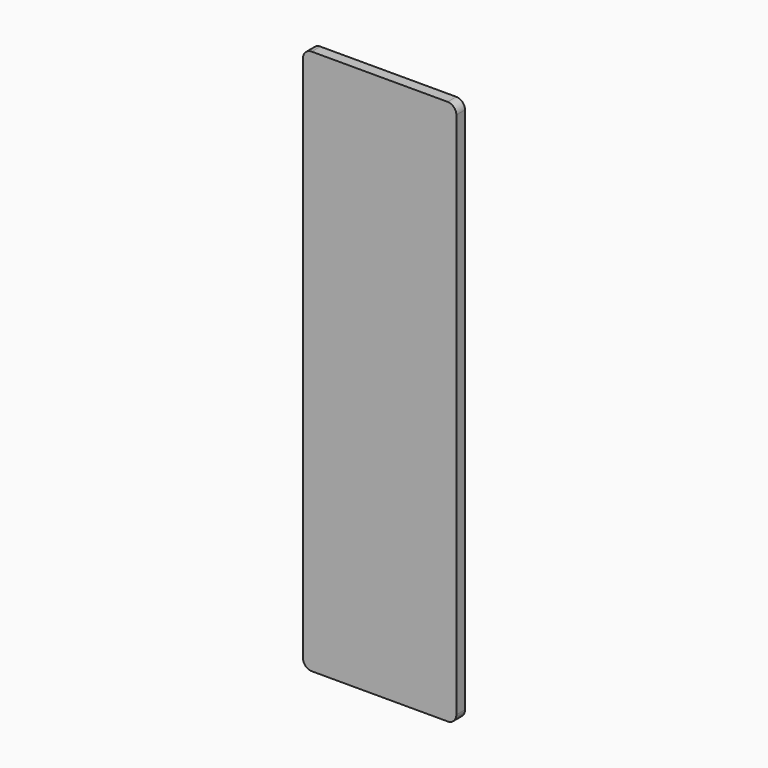
from build123d import *

# Parameters (mm, degrees)
F1_DEPTH = 3.175


# Not quite as in the source:
# - a length typed as a fraction of an inch, garbled in the dataset ("3 / 203.2 mm" for 3/8 in), is restored


with BuildPart() as f1:
    # F0 (on Front) → F1 (new body)
    with BuildSketch(Plane.XZ):
        with BuildLine():
            Line((21.49735579, 94.8843865406), (-18.12664421, 94.8843865406))
            ThreePointArc((-18.12664421, 94.8843865406), (-19.9226954343, 94.1404377648), (-20.66664421, 92.3443865406))
            Line((-20.66664421, 92.3443865406), (-20.66664421, -61.5796134594))
            ThreePointArc((-20.66664421, -61.5796134594), (-19.9226954343, -63.3756646836), (-18.12664421, -64.1196134594))
            Line((-18.12664421, -64.1196134594), (21.49735579, -64.1196134594))
            ThreePointArc((21.49735579, -64.1196134594), (23.2934070142, -63.3756646836), (24.03735579, -61.5796134594))
            Line((24.03735579, -61.5796134594), (24.03735579, 92.3443865406))
            ThreePointArc((24.03735579, 92.3443865406), (23.2934070142, 94.1404377648), (21.49735579, 94.8843865406))
        make_face()
    extrude(amount=F1_DEPTH)


solid = f1.part
